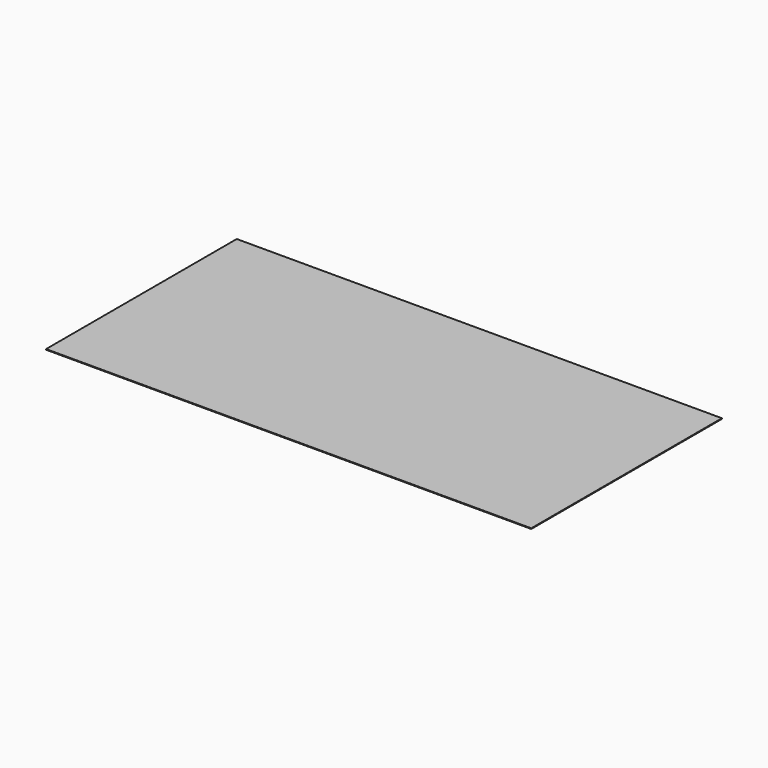
from build123d import *

# Parameters (mm, degrees)
F0_W     = 80.9329524636
F0_H     = 39.7536940873
F1_DEPTH = 0.109


with BuildPart() as f1:
    # F0 (on Top) → F1 (new body)
    with BuildSketch(Plane.XY):
        with Locations((16.0759501159, 1.0920297354)):
            Rectangle(F0_W, F0_H)
    extrude(amount=F1_DEPTH)


with BuildPart() as f1_1:
    # F2: moved
    add(f1.part.moved(Location((80.9329524636, 0, 0))))


solid = f1_1.part
